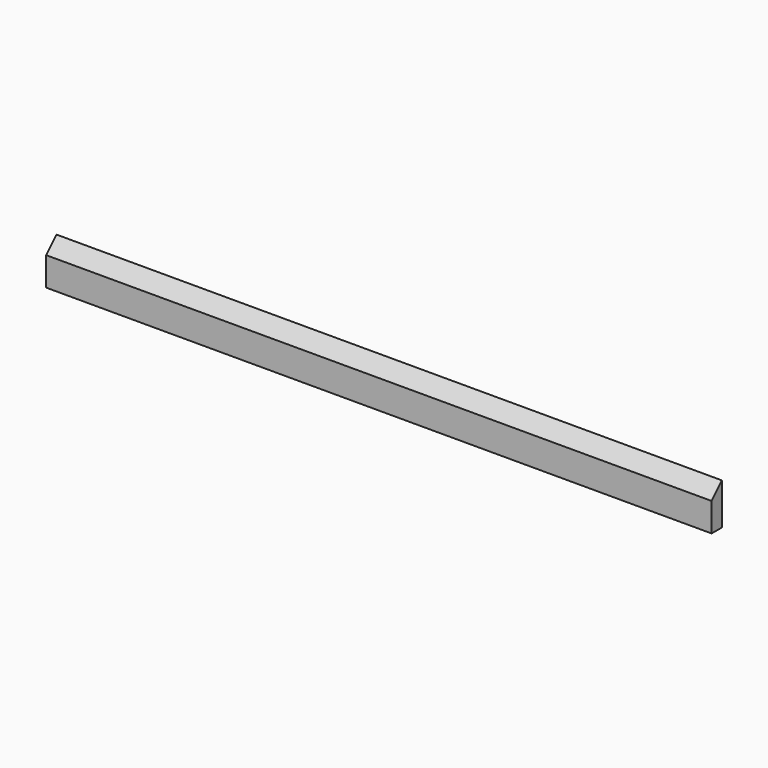
from build123d import *

# Parameters (mm, degrees)
F0_W     = 930
F0_H     = 58
F1_DEPTH = 18
F2_SIZE  = 17.99999


# Not quite as in the source:
# - a fillet or chamfer is up to 0.001 mm smaller than in the source, because OpenCascade refuses the exact size


with BuildPart() as f1:
    # F0 (on Front) → F1 (new body)
    with BuildSketch(Plane.XZ):
        Rectangle(F0_W, F0_H)
    extrude(amount=F1_DEPTH)

    # F2 (size 18 in the source; OpenCascade refuses exactly that, so slightly less here)
    f2_edges = [f1.edges().sort_by_distance(p)[0] for p in [
        (0, -18, 29),
    ]]
    chamfer(f2_edges, length=F2_SIZE)


solid = f1.part
